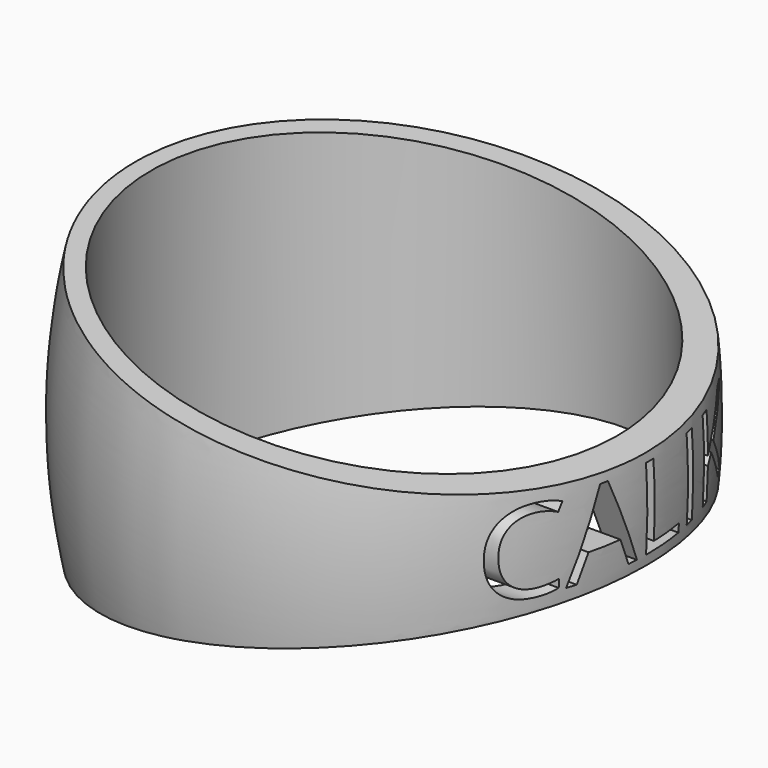
from build123d import *

# Parameters (mm, degrees)
F4_DEPTH     = 35
F6_TEXT_SIZE = 7.2988538519
F7_DEPTH     = 7


# Not quite as in the source:
# - Text() gives the source's letters only with a copy of the font that has no kerning and outlines rounded to 1/6400 em; it was checked with that copy


with BuildPart() as f1:
    # F0 (on Front) → F1 (revolve)
    with BuildSketch(Plane.XZ):
        with BuildLine():
            Line((15, -9), (16, -9))
            ThreePointArc((16, -9), (17, 0), (16, 9))
            Line((16, 9), (15, 9))
            Line((15, 9), (15, -9))
        make_face()
    revolve(axis=Axis((0, 0, -2.4727410637), (0, 0, -1)))

    # F3 (on offset) → F4 (cut)
    with BuildSketch(Plane.XZ.offset(17)):
        Polygon((16, 9), (-16, 9), (18.4682713554, 2.9223137817), align=None)
        Polygon((18.4682713554, -2.9223137817), (-16, -9), (16, -9), align=None)
    extrude(amount=-F4_DEPTH, mode=Mode.SUBTRACT)

    # F6 (on offset) → F7 (cut)
    with BuildSketch(Plane.YZ.offset(17)):
        with Locations((-10, -2.5602408776)):
            Text('CALIK', F6_TEXT_SIZE, font='Open Sans', text_align=(TextAlign.LEFT, TextAlign.BOTTOM))
        with BuildLine():
            Line((-3.9259850602, -0.358039817), (-2.2404059987, -0.358039817))
            Line((-2.2404059987, -0.358039817), (-2.8471232252, 1.2568315977))
            add(Edge.make_bspline(
                [(-2.8471232252, 1.2568315977), (-2.9645891544, 1.5636115487), (-3.088897759, 2.0083854553)],
                knots=[0, 0, 0, 1, 1, 1], degree=2))
            add(Edge.make_bspline(
                [(-3.088897759, 2.0083854553), (-3.1675885271, 1.666251681), (-3.3135656042, 1.2568315977)],
                knots=[0, 0, 0, 1, 1, 1], degree=2))
            Line((-3.3135656042, 1.2568315977), (-3.9259850602, -0.358039817))
        make_face()
    extrude(amount=-F7_DEPTH, mode=Mode.SUBTRACT)


solid = f1.part
